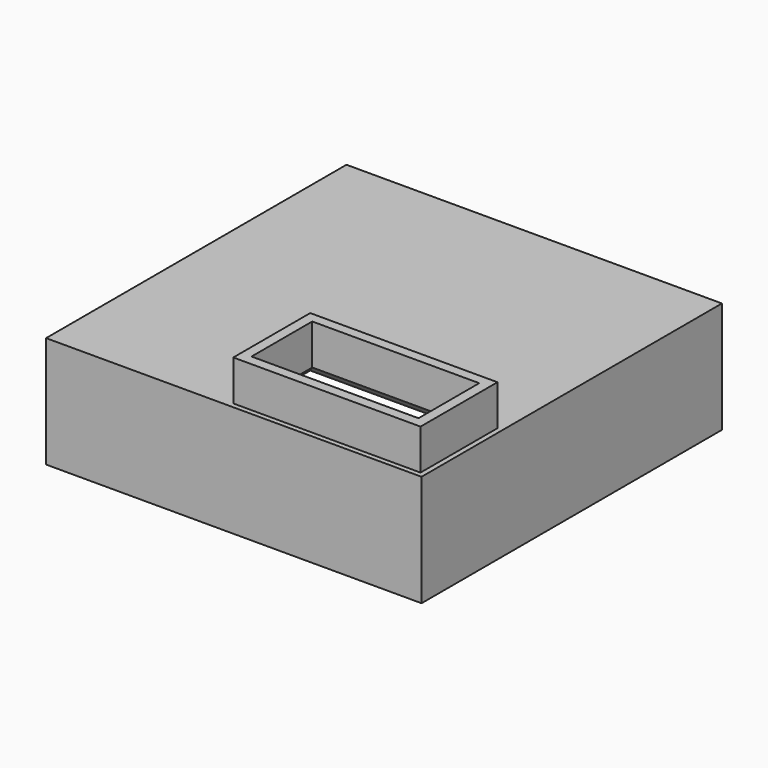
from build123d import *

# Parameters (mm, degrees)
F0_W          = 70.2
F0_H          = 70.2
F1_DEPTH      = 20
F2_T          = 2
F3_W          = 33
F3_H          = 15
F4_DEPTH      = 25
F5_DEPTH      = 25
F6_T          = 2
F7_W          = 2
F7_H          = 6.9346216321
F7_W_2        = 33
F7_H_2        = 10.0653783679
F8_DEPTH      = 25
F9_T1_DEPTH   = 70.2
F9_T3_DEPTH   = 70.2
F9_T8_DEPTH   = 70.2
F9_T14_DEPTH  = 70.2
F9_T20_DEPTH  = 70.2
F9_T27_DEPTH  = 70.2
F9_T33_DEPTH  = 70.2
F9_T39_DEPTH  = 70.2
F9_T45_DEPTH  = 70.2
F9_T51_DEPTH  = 70.2
F9_T58_DEPTH  = 70.2
F9_T64_DEPTH  = 70.2
F10_T1_DEPTH  = 25.0674098192
F10_T6_ANGLE  = 95.6264745755
F10_T11_ANGLE = 95.6264745755
F10_T16_DEPTH = 14.2107757951


# Not quite as in the source:
# - a fillet or chamfer that OpenCascade refuses, or shapes differently, is made with other operations: its cross-section is extruded or revolved along the edge and cut away or added


with BuildPart() as f1:
    # F0 (on Top) → F1 (new body)
    with BuildSketch(Plane.XY):
        Rectangle(F0_W, F0_H)
    extrude(amount=F1_DEPTH)

    # F2
    f2_openings = [f1.faces().sort_by_distance(p)[0] for p in [
        (0, 0, 0),
    ]]
    offset(amount=F2_T, openings=f2_openings, kind=Kind.INTERSECTION)

    # F3 (on face) → F4 (cut)
    with BuildSketch(Plane.XY.offset(22)):
        with Locations((17.6, -26.6)):
            Rectangle(F3_W, F3_H)
    extrude(amount=-F4_DEPTH, mode=Mode.SUBTRACT)

    # F9: fillet of radius 8.9325901808 on 4 edges, made by hand

    # F9_s2 → F9_t1 (join)
    with BuildSketch(Plane.YZ.offset(-35.1)):
        with BuildLine():
            ThreePointArc((35.1, 11.0674098192), (32.4837049096, 17.3837049096), (26.1674098192, 20))
            Line((26.1674098192, 20), (35.1, 20))
            Line((35.1, 20), (35.1, 11.0674098192))
        make_face()
    extrude(amount=F9_T1_DEPTH)

    # F9_s4 → F9_t3 (join)
    with BuildSketch(Plane.XZ.offset(-35.1)):
        with BuildLine():
            ThreePointArc((-35.1, 11.0674098192), (-32.4837049096, 17.3837049096), (-26.1674098192, 20))
            Line((-26.1674098192, 20), (-35.1, 20))
            Line((-35.1, 20), (-35.1, 11.0674098192))
        make_face()
    extrude(amount=F9_T3_DEPTH)


with BuildPart() as f5:
    # F3 (on face) → F5 (new body)
    with BuildSketch(Plane.XY.offset(22)):
        with Locations((17.6, -26.6)):
            Rectangle(F3_W, F3_H)
    extrude(amount=F5_DEPTH)

    # F6
    f6_openings = [f5.faces().sort_by_distance(p)[0] for p in [
        (17.6, -26.6, 22),
    ]]
    offset(amount=F6_T, openings=f6_openings, kind=Kind.INTERSECTION)

    # F7 (on face) → F8 (cut)
    with BuildSketch(Plane.XZ.offset(36.1)):
        with Locations((0.1, 33.467310816)):
            Rectangle(F7_W, F7_H)
        with Locations((17.6, 33.467310816)):
            Rectangle(F7_W_2, F7_H)
        Polygon((-0.9, 49), (-0.9, 36.9346216321), (1.1, 36.9346216321), (1.1, 47), (34.1, 47), (34.1, 36.9346216321), (36.1, 36.9346216321), (36.1, 49), align=None)
        with Locations((35.1, 33.467310816)):
            Rectangle(F7_W, F7_H)
        with Locations((17.6, 41.967310816)):
            Rectangle(F7_W_2, F7_H_2)
    extrude(amount=-F8_DEPTH, mode=Mode.SUBTRACT)


with BuildPart() as f9_tool6:
    # F9_s7 → F9_t8 (new body)
    with BuildSketch(Plane.XZ.offset(35.1)):
        with BuildLine():
            ThreePointArc((35.1, 11.0674098192), (32.4837049096, 17.3837049096), (26.1674098192, 20))
            Line((26.1674098192, 20), (35.1, 20))
            Line((35.1, 20), (35.1, 11.0674098192))
        make_face()
    extrude(amount=-F9_T8_DEPTH)

    split(bisect_by=Plane.XZ.offset(34.1), keep=Keep.TOP)

    split(bisect_by=Plane.YZ.offset(34.1), keep=Keep.TOP)


with BuildPart() as f1_1:
    add(f1.part)

    # F9_t5: union F9_tool6
    add(f9_tool6.part)


with BuildPart() as f9_tool12:
    # F9_s13 → F9_t14 (new body)
    with BuildSketch(Plane.XZ.offset(35.1)):
        with BuildLine():
            ThreePointArc((35.1, 11.0674098192), (32.4837049096, 17.3837049096), (26.1674098192, 20))
            Line((26.1674098192, 20), (35.1, 20))
            Line((35.1, 20), (35.1, 11.0674098192))
        make_face()
    extrude(amount=-F9_T14_DEPTH)

    split(bisect_by=Plane.XZ.offset(34.1), keep=Keep.TOP)

    split(bisect_by=Plane.YZ.offset(34.1), keep=Keep.BOTTOM)


with BuildPart() as f1_2:
    add(f1_1.part)

    # F9_t11: union F9_tool12
    add(f9_tool12.part)


with BuildPart() as f9_tool18:
    # F9_s19 → F9_t20 (new body)
    with BuildSketch(Plane.XZ.offset(35.1)):
        with BuildLine():
            ThreePointArc((35.1, 11.0674098192), (32.4837049096, 17.3837049096), (26.1674098192, 20))
            Line((26.1674098192, 20), (35.1, 20))
            Line((35.1, 20), (35.1, 11.0674098192))
        make_face()
    extrude(amount=-F9_T20_DEPTH)

    split(bisect_by=Plane.XZ.offset(19.1), keep=Keep.TOP)

    split(bisect_by=Plane.XZ.offset(34.1), keep=Keep.BOTTOM)

    split(bisect_by=Plane.YZ.offset(34.1), keep=Keep.TOP)


with BuildPart() as f1_3:
    add(f1_2.part)

    # F9_t17: union F9_tool18
    add(f9_tool18.part)


with BuildPart() as f9_tool25:
    # F9_s26 → F9_t27 (new body)
    with BuildSketch(Plane.XZ.offset(35.1)):
        with BuildLine():
            ThreePointArc((35.1, 11.0674098192), (32.4837049096, 17.3837049096), (26.1674098192, 20))
            Line((26.1674098192, 20), (35.1, 20))
            Line((35.1, 20), (35.1, 11.0674098192))
        make_face()
    extrude(amount=-F9_T27_DEPTH)

    split(bisect_by=Plane.XZ.offset(19.1), keep=Keep.BOTTOM)

    split(bisect_by=Plane.YZ.offset(34.1), keep=Keep.TOP)


with BuildPart() as f1_4:
    add(f1_3.part)

    # F9_t24: union F9_tool25
    add(f9_tool25.part)


with BuildPart() as f9_tool31:
    # F9_s32 → F9_t33 (new body)
    with BuildSketch(Plane.XZ.offset(35.1)):
        with BuildLine():
            ThreePointArc((35.1, 11.0674098192), (32.4837049096, 17.3837049096), (26.1674098192, 20))
            Line((26.1674098192, 20), (35.1, 20))
            Line((35.1, 20), (35.1, 11.0674098192))
        make_face()
    extrude(amount=-F9_T33_DEPTH)

    split(bisect_by=Plane.XZ.offset(19.1), keep=Keep.BOTTOM)

    split(bisect_by=Plane.YZ.offset(34.1), keep=Keep.BOTTOM)


with BuildPart() as f1_5:
    add(f1_4.part)

    # F9_t30: union F9_tool31
    add(f9_tool31.part)


with BuildPart() as f9_tool37:
    # F9_s38 → F9_t39 (new body)
    with BuildSketch(Plane.YZ.offset(-35.1)):
        with BuildLine():
            ThreePointArc((-26.1674098192, 20), (-32.4837049096, 17.3837049096), (-35.1, 11.0674098192))
            Line((-35.1, 11.0674098192), (-35.1, 20))
            Line((-35.1, 20), (-26.1674098192, 20))
        make_face()
    extrude(amount=F9_T39_DEPTH)

    split(bisect_by=Plane.YZ.offset(1.1), keep=Keep.BOTTOM)

    split(bisect_by=Plane.XZ.offset(34.1), keep=Keep.BOTTOM)


with BuildPart() as f1_6:
    add(f1_5.part)

    # F9_t36: union F9_tool37
    add(f9_tool37.part)


with BuildPart() as f9_tool43:
    # F9_s44 → F9_t45 (new body)
    with BuildSketch(Plane.YZ.offset(-35.1)):
        with BuildLine():
            ThreePointArc((-26.1674098192, 20), (-32.4837049096, 17.3837049096), (-35.1, 11.0674098192))
            Line((-35.1, 11.0674098192), (-35.1, 20))
            Line((-35.1, 20), (-26.1674098192, 20))
        make_face()
    extrude(amount=F9_T45_DEPTH)

    split(bisect_by=Plane.YZ.offset(1.1), keep=Keep.BOTTOM)

    split(bisect_by=Plane.XZ.offset(34.1), keep=Keep.TOP)


with BuildPart() as f1_7:
    add(f1_6.part)

    # F9_t42: union F9_tool43
    add(f9_tool43.part)


with BuildPart() as f9_tool49:
    # F9_s50 → F9_t51 (new body)
    with BuildSketch(Plane.YZ.offset(-35.1)):
        with BuildLine():
            ThreePointArc((-26.1674098192, 20), (-32.4837049096, 17.3837049096), (-35.1, 11.0674098192))
            Line((-35.1, 11.0674098192), (-35.1, 20))
            Line((-35.1, 20), (-26.1674098192, 20))
        make_face()
    extrude(amount=F9_T51_DEPTH)

    split(bisect_by=Plane.YZ.offset(1.1), keep=Keep.TOP)

    split(bisect_by=Plane.XZ.offset(34.1), keep=Keep.TOP)

    split(bisect_by=Plane.YZ.offset(34.1), keep=Keep.BOTTOM)


with BuildPart() as f1_8:
    add(f1_7.part)

    # F9_t48: union F9_tool49
    add(f9_tool49.part)


with BuildPart() as f9_tool56:
    # F9_s57 → F9_t58 (new body)
    with BuildSketch(Plane.YZ.offset(-35.1)):
        with BuildLine():
            ThreePointArc((-26.1674098192, 20), (-32.4837049096, 17.3837049096), (-35.1, 11.0674098192))
            Line((-35.1, 11.0674098192), (-35.1, 20))
            Line((-35.1, 20), (-26.1674098192, 20))
        make_face()
    extrude(amount=F9_T58_DEPTH)

    split(bisect_by=Plane.XZ.offset(34.1), keep=Keep.BOTTOM)

    split(bisect_by=Plane.YZ.offset(34.1), keep=Keep.TOP)


with BuildPart() as f1_9:
    add(f1_8.part)

    # F9_t55: union F9_tool56
    add(f9_tool56.part)


with BuildPart() as f9_tool62:
    # F9_s63 → F9_t64 (new body)
    with BuildSketch(Plane.YZ.offset(-35.1)):
        with BuildLine():
            ThreePointArc((-26.1674098192, 20), (-32.4837049096, 17.3837049096), (-35.1, 11.0674098192))
            Line((-35.1, 11.0674098192), (-35.1, 20))
            Line((-35.1, 20), (-26.1674098192, 20))
        make_face()
    extrude(amount=F9_T64_DEPTH)

    split(bisect_by=Plane.XZ.offset(34.1), keep=Keep.TOP)

    split(bisect_by=Plane.YZ.offset(34.1), keep=Keep.TOP)


with BuildPart() as f1_10:
    add(f1_9.part)

    # F9_t61: union F9_tool62
    add(f9_tool62.part)

    # F10: chamfer of 2 on 6 edges, made by hand

    # F10_s2 → F10_t1 (cut)
    with BuildSketch(Plane.YZ.offset(1.1)):
        Polygon((-17.1, 20), (-19.1, 22), (-19.1, 20), align=None)
    extrude(amount=F10_T1_DEPTH, mode=Mode.SUBTRACT)


with BuildPart() as f10_tool4:
    # F10_s5 → F10_t6 (revolve)
    with BuildSketch(Plane(origin=(1.331382753, 0, 13.5141903658), x_dir=(0, 1, 0), z_dir=(-0.0980427526, 0, -0.9951822038))):
        Polygon((-17.1, 33.8888514287), (-19.1, 35.8888514287), (-19.1, 33.8888514287), align=None)
    revolve(axis=Axis((26.1674098192, -19.1, 11.0674098192), (0, -1, 0)), revolution_arc=F10_T6_ANGLE)

    split(bisect_by=Plane.YZ.offset(34.1), keep=Keep.BOTTOM)


with BuildPart() as f1_11:
    add(f1_10.part)

    # F10_t3: cut F10_tool4
    add(f10_tool4.part, mode=Mode.SUBTRACT)


with BuildPart() as f10_tool9:
    # F10_s10 → F10_t11 (revolve)
    with BuildSketch(Plane(origin=(0, -1.331382753, 13.5141903658), x_dir=(1, 0, 0), z_dir=(0, 0.0980427526, -0.9951822038))):
        Polygon((1.1, 35.8888514287), (-0.9, 33.8888514287), (1.1, 33.8888514287), align=None)
    revolve(axis=Axis((1.1, -26.1674098192, 11.0674098192), (-1, 0, 0)), revolution_arc=F10_T11_ANGLE)

    split(bisect_by=Plane.XZ.offset(34.1), keep=Keep.BOTTOM)


with BuildPart() as f1_12:
    add(f1_11.part)

    # F10_t8: cut F10_tool9
    add(f10_tool9.part, mode=Mode.SUBTRACT)


with BuildPart() as f10_tool14:
    # F10_s15 → F10_t16 (new body)
    with BuildSketch(Plane.XZ.offset(11.9566340241)):
        Polygon((-0.9, 20), (1.1, 22), (1.1, 20), align=None)
    extrude(amount=F10_T16_DEPTH)

    split(bisect_by=Plane(origin=(0, 1.45, 1.45), x_dir=(1, 0, 0), z_dir=(0, -0.7071067812, -0.7071067812)), keep=Keep.TOP)


with BuildPart() as f1_13:
    add(f1_12.part)

    # F10_t13: cut F10_tool14
    add(f10_tool14.part, mode=Mode.SUBTRACT)


solid = Compound([f5.part, f1_13.part])
